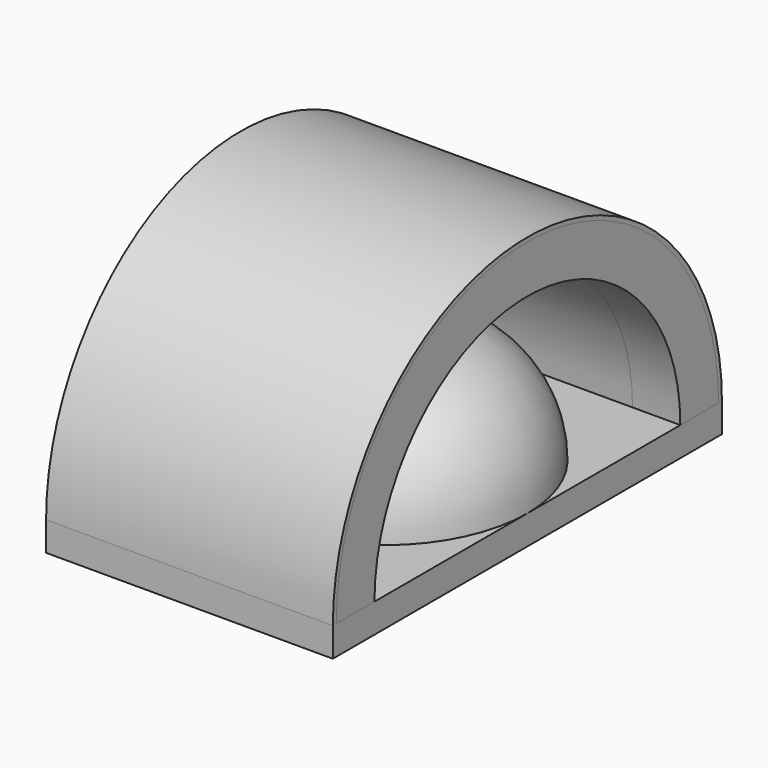
from build123d import *

# Parameters (mm, degrees)
F0_R          = 30
F1_DEPTH      = 25
F2_R          = 24.99999
F4_DEPTH      = 30
F4_DEPTH_BACK = 30
F5_DEPTH      = 30
F5_DEPTH_BACK = 30
F6_R          = 10


# Not quite as in the source:
# - a fillet or chamfer is up to 0.001 mm smaller than in the source, because OpenCascade refuses the exact size


with BuildPart() as f1:
    # F0 (on Top) → F1 (new body)
    with BuildSketch(Plane.XY):
        Circle(F0_R)
    extrude(amount=F1_DEPTH)

    # F2 (radius 25 in the source; OpenCascade refuses exactly that, so slightly less here)
    f2_edges = [f1.edges().sort_by_distance(p)[0] for p in [
        (-30, 0, 25),
    ]]
    fillet(f2_edges, radius=F2_R)


with BuildPart() as f4:
    # F3 (on Right) → F4 (new body, two sides)
    with BuildSketch(Plane.YZ) as f4_sk:
        with BuildLine():
            ThreePointArc((50.8803409753, 0), (0, 50.8803409753), (-50.8803409753, 0))
            Line((-50.8803409753, 0), (-40, 0))
            ThreePointArc((-40, 0), (0, 40), (40, 0))
            Line((40, 0), (50.8803409753, 0))
        make_face()
    extrude(amount=F4_DEPTH)
    extrude(f4_sk.sketch, amount=-F4_DEPTH_BACK)


with BuildPart() as f5:
    # F3 (on Right) → F5 (new body, two sides)
    with BuildSketch(Plane.YZ) as f5_sk:
        with BuildLine():
            ThreePointArc((50.8803409753, 0), (0, 50.8803409753), (-50.8803409753, 0))
            Line((-50.8803409753, 0), (-40, 0))
            ThreePointArc((-40, 0), (0, 40), (40, 0))
            Line((40, 0), (50.8803409753, 0))
        make_face()
        Polygon((-40, 0), (-50.8803409753, 0), (-50.8803409753, -6.0972881854), (50.8803409753, -6.0972881854), (50.8803409753, 0), (40, 0), align=None)
    extrude(amount=F5_DEPTH)
    extrude(f5_sk.sketch, amount=-F5_DEPTH_BACK)

    # F6
    f6_edges = [f5.edges().sort_by_distance(p)[0] for p in [
        (30, 0, 40),
    ]]
    fillet(f6_edges, radius=F6_R)


solid = Compound([f1.part, f4.part, f5.part])
